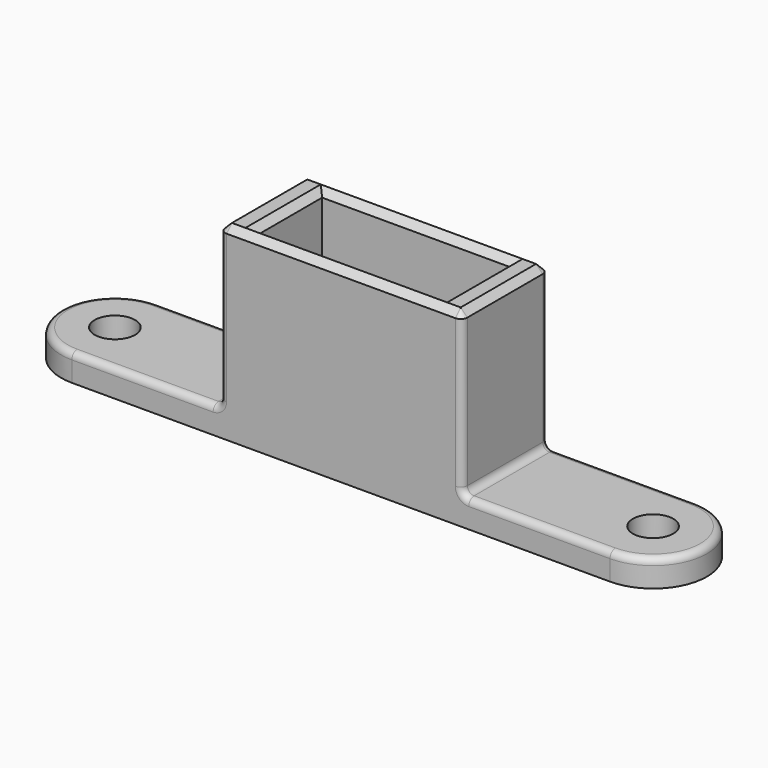
from build123d import *

# Parameters (mm, degrees)
F0_R          = 1.5
F1_DEPTH      = 2
F2_W          = 18
F2_H          = 8
F2_W_2        = 14
F2_H_2        = 6
F3_DEPTH      = 14
F4_R          = 0.5
F5_SIZE       = 0.49999
F6_W          = 14
F6_H          = 6
F7_DEPTH      = 2.001
F8_W          = 17
F8_H          = 2
F9_DEPTH      = 3
F9_DEPTH_BACK = 3
F10_W         = 1
F10_H         = 6
F11_DEPTH     = 1
F12_R         = 0.25
F13_DEPTH     = 6.001
F14_W         = 14
F14_H         = 1
F15_DEPTH     = 4


# Not quite as in the source:
# - a fillet or chamfer is up to 0.001 mm smaller than in the source, because OpenCascade refuses the exact size


with BuildPart() as f1:
    # F0 (on Top) → F1 (new body)
    with BuildSketch(Plane.XY):
        with BuildLine():
            Line((20, 4), (0, 4))
            Line((0, 4), (-20, 4))
            ThreePointArc((-20, 4), (-24, 0), (-20, -4))
            Line((-20, -4), (0, -4))
            Line((0, -4), (20, -4))
            ThreePointArc((20, -4), (24, 0), (20, 4))
        make_face()
        with Locations((-20, 0)):
            Circle(F0_R, mode=Mode.SUBTRACT)
        with Locations((20, 0)):
            Circle(F0_R, mode=Mode.SUBTRACT)
    extrude(amount=F1_DEPTH)

    # F2 (on Top) → F3 (join)
    with BuildSketch(Plane.XY):
        Rectangle(F2_W, F2_H)
        Rectangle(F2_W_2, F2_H_2, mode=Mode.SUBTRACT)
    extrude(amount=F3_DEPTH)

    # F4
    f4_edges = [f1.edges().sort_by_distance(p)[0] for p in [
        (9, 0, 2),
        (-9, 0, 2),
        (-9, -4, 8),
        (9, -4, 8),
        (24, 0, 2),
        (14.5, -4, 2),
        (14.5, 4, 2),
        (9, 4, 8),
        (-9, 4, 8),
        (-14.5, -4, 2),
        (-24, 0, 2),
        (-14.5, 4, 2),
    ]]
    fillet(f4_edges, radius=F4_R)

    # F5 (size 0.5 in the source; OpenCascade refuses exactly that, so slightly less here)
    f5_edges = [f1.edges().sort_by_distance(p)[0] for p in [
        (7, 0, 14),
        (0, 3, 14),
        (-7, 0, 14),
        (0, -3, 14),
        (0, -4, 14),
        (0, 4, 14),
        (-8.853553, -3.853553, 14),
        (8.853553, -3.853553, 14),
        (-9, 0, 14),
        (9, 0, 14),
        (-8.853553, 3.853553, 14),
        (8.853553, 3.853553, 14),
    ]]
    chamfer(f5_edges, length=F5_SIZE)

    # F6 (on face) → F7 (cut, through all)
    with BuildSketch(Plane.XY.offset(2)):
        Rectangle(F6_W, F6_H)
    extrude(amount=-F7_DEPTH, mode=Mode.SUBTRACT)

    # F8 (on Front) → F9 (join, two sides)
    with BuildSketch(Plane.XZ) as f9_sk:
        with Locations((0, 5)):
            Rectangle(F8_W, F8_H)
    extrude(amount=-F9_DEPTH)
    extrude(f9_sk.sketch, amount=F9_DEPTH_BACK)

    # F10 (on face) → F11 (join)
    with BuildSketch(Plane.XY.offset(6)):
        with Locations((1.5, 0)):
            Rectangle(F10_W, F10_H)
        with Locations((-4.5, 0)):
            Rectangle(F10_W, F10_H)
    extrude(amount=F11_DEPTH)

    # F12 (on face) → F13 (cut, through all)
    with BuildSketch(Plane.XY.offset(6)):
        with Locations((-2, 1)):
            Circle(F12_R)
        with Locations((-2, -1)):
            Circle(F12_R)
        with Locations((4, 1)):
            Circle(F12_R)
        with Locations((4, -1)):
            Circle(F12_R)
        with Locations((-6, 1)):
            Circle(F12_R)
        with Locations((-6, -1)):
            Circle(F12_R)
    extrude(amount=-F13_DEPTH, mode=Mode.SUBTRACT)

    # F14 (on face) → F15 (join, through all)
    with BuildSketch(Plane(origin=(0, 0, 4), x_dir=(1, 0, 0), z_dir=(0, 0, -1))):
        with Locations((0, -0.056592231)):
            Rectangle(F14_W, F14_H)
    extrude(amount=F15_DEPTH)


solid = f1.part
